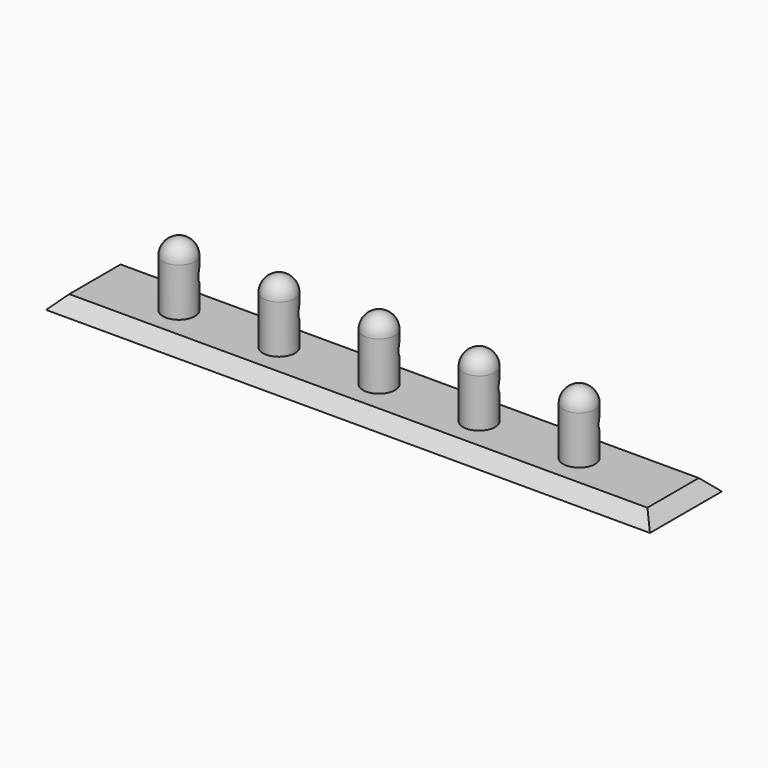
from build123d import *

# Parameters (mm, degrees)
F0_W        = 190
F0_H        = 30
F1_DEPTH    = 4
F2_R        = 5
F3_DEPTH    = 20
F4_R        = 5.25
F5_DEPTH    = 2.3
F6_T1_DEPTH = 215.7168298797
F6_T3_DEPTH = 55.7168298797
F7_R        = 2.75
F8_DEPTH    = 75
F9_R        = 5


# Not quite as in the source:
# - a fillet or chamfer that OpenCascade refuses, or shapes differently, is made with other operations: its cross-section is extruded or revolved along the edge and cut away or added


with BuildPart() as f1:
    # F0 (on Top) → F1 (new body)
    with BuildSketch(Plane.XY):
        with Locations((1.5441179276, 0)):
            Rectangle(F0_W, F0_H)
    extrude(amount=-F1_DEPTH)

    # F2 (on Top) → F3 (join)
    with BuildSketch(Plane.XY):
        with Locations((-62.3, 0)):
            Circle(F2_R)
        with Locations((-31.15, 0)):
            Circle(F2_R)
        Circle(F2_R)
        with Locations((31.15, 0)):
            Circle(F2_R)
        with Locations((62.3, 0)):
            Circle(F2_R)
    extrude(amount=F3_DEPTH)

    # F4 (on face) → F5 (cut)
    with BuildSketch(Plane(origin=(0, 0, -4), x_dir=(1, 0, 0), z_dir=(0, 0, -1))):
        with Locations((-75, 0)):
            Circle(F4_R)
        Circle(F4_R)
        with Locations((75, 0)):
            Circle(F4_R)
    extrude(amount=-F5_DEPTH, mode=Mode.SUBTRACT)

    # F6: chamfer of 5 on 4 edges, made by hand

    # F6_s2 → F6_t1 (cut)
    with BuildSketch(Plane.YZ.offset(-106.3142970123)):
        Polygon((15, -5), (10, 0), (15, 0), align=None)
        Polygon((-10, 0), (-15, -5), (-15, 0), align=None)
    extrude(amount=F6_T1_DEPTH, mode=Mode.SUBTRACT)

    # F6_s4 → F6_t3 (cut)
    with BuildSketch(Plane.XZ.offset(-27.8584149398)):
        Polygon((96.5441179276, -5), (91.5441179276, 0), (96.5441179276, 0), align=None)
        Polygon((-93.4558820724, -5), (-88.4558820724, 0), (-93.4558820724, 0), align=None)
    extrude(amount=F6_T3_DEPTH, mode=Mode.SUBTRACT)

    # F7 (on Right) → F8 (cut, symmetric)
    with BuildSketch(Plane.YZ):
        with Locations((4.4393371791, 10)):
            Circle(F7_R)
    extrude(amount=F8_DEPTH, both=True, mode=Mode.SUBTRACT)

    # F9
    f9_edges = [f1.edges().sort_by_distance(p)[0] for p in [
        (-67.3, 0, 20),
        (-36.15, 0, 20),
        (-5, 0, 20),
        (26.15, 0, 20),
        (57.3, 0, 20),
    ]]
    fillet(f9_edges, radius=F9_R)


solid = f1.part
